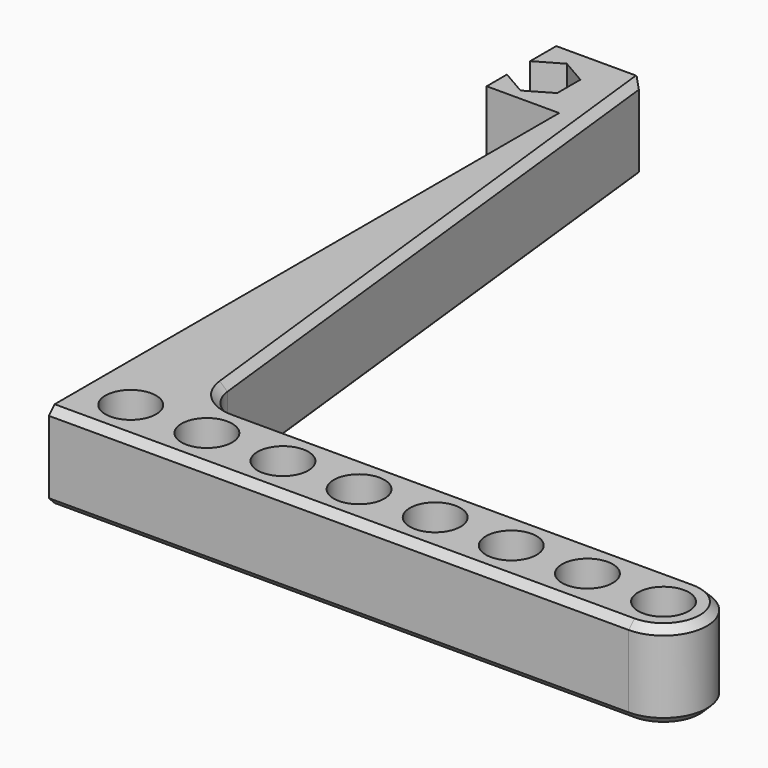
from build123d import *

# Parameters (mm, degrees)
F0_R         = 3.5
F1_DEPTH     = 12
F3_DEPTH     = 25
F4_R         = 5
F5_W         = 12
F5_H         = 12
F6_DEPTH     = 10
F8_T1_DEPTH  = 86.6740446023
F8_T3_DEPTH  = 16.6151120325
F8_T5_DEPTH  = 82.571682988
F8_T7_DEPTH  = 63.5360023124
F8_T10_ANGLE = 180
F8_T12_ANGLE = 83.5169263071
F8_T14_ANGLE = 180
F8_T16_ANGLE = 83.5169263071
F9_DEPTH     = 25


# Not quite as in the source:
# - a fillet or chamfer that OpenCascade refuses, or shapes differently, is made with other operations: its cross-section is extruded or revolved along the edge and cut away or added


with BuildPart() as f1:
    # F0 (on Top) → F1 (new body)
    with BuildSketch(Plane.XY):
        with BuildLine():
            Line((12, 100), (0, 100))
            Line((0, 100), (0, 0))
            Line((0, 0), (80, 0))
            ThreePointArc((80, 0), (86, 6), (80, 12))
            Line((80, 12), (12, 12))
            Line((12, 12), (12, 100))
        make_face()
        with Locations((6.5, 6)):
            Circle(F0_R, mode=Mode.SUBTRACT)
        with Locations((17, 6)):
            Circle(F0_R, mode=Mode.SUBTRACT)
        with Locations((27.5, 6)):
            Circle(F0_R, mode=Mode.SUBTRACT)
        with Locations((38, 6)):
            Circle(F0_R, mode=Mode.SUBTRACT)
        with Locations((48.5, 6)):
            Circle(F0_R, mode=Mode.SUBTRACT)
        with Locations((59, 6)):
            Circle(F0_R, mode=Mode.SUBTRACT)
        with Locations((69.5, 6)):
            Circle(F0_R, mode=Mode.SUBTRACT)
        with Locations((80, 6)):
            Circle(F0_R, mode=Mode.SUBTRACT)
    extrude(amount=F1_DEPTH)

    # F2 (on face) → F3 (cut)
    with BuildSketch(Plane.XY.offset(12)):
        Polygon((2, 100), (12, 12), (12, 100), align=None)
    extrude(amount=-F3_DEPTH, mode=Mode.SUBTRACT)

    # F4
    f4_edges = [f1.edges().sort_by_distance(p)[0] for p in [
        (12, 12, 6),
    ]]
    fillet(f4_edges, radius=F4_R)

    # F5 (on face) → F6 (join)
    with BuildSketch(Plane(origin=(0, 0, 0), x_dir=(0, -1, 0), z_dir=(-1, 0, 0))):
        with Locations((-94, 6)):
            Rectangle(F5_W, F5_H)
    extrude(amount=F6_DEPTH)

    # F8: chamfer of 1 on 11 edges, made by hand

    # F8_s2 → F8_t1 (cut)
    with BuildSketch(Plane(origin=(-11.4836366644, 101.0560026464, 0), x_dir=(0, 0, 1), z_dir=(0.112909688, -0.9936052548, 0))):
        Polygon((12, -12.278179314), (11, -13.278179314), (12, -13.278179314), align=None)
        Polygon((0, -12.278179314), (1, -13.278179314), (0, -13.278179314), align=None)
    extrude(amount=F8_T1_DEPTH, mode=Mode.SUBTRACT)

    # F8_s4 → F8_t3 (cut)
    with BuildSketch(Plane.XY.offset(-2.3075560163)):
        Polygon((1.1072004625, 100), (2.1008057173, 99.112909688), (2, 100), align=None)
    extrude(amount=F8_T3_DEPTH, mode=Mode.SUBTRACT)

    # F8_s6 → F8_t5 (cut)
    with BuildSketch(Plane.YZ.offset(-2.571682988)):
        Polygon((1, 0), (0, 1), (0, 0), align=None)
        Polygon((1, 12), (0, 11), (0, 12), align=None)
    extrude(amount=F8_T5_DEPTH, mode=Mode.SUBTRACT)

    # F8_s8 → F8_t7 (cut)
    with BuildSketch(Plane.YZ.offset(16.4639976876)):
        Polygon((11, 0), (12, 1), (12, 0), align=None)
        Polygon((11, 12), (12, 11), (12, 12), align=None)
    extrude(amount=F8_T7_DEPTH, mode=Mode.SUBTRACT)

    # F8_s9 → F8_t10 (revolve, cut)
    with BuildSketch(Plane.YZ.offset(80)):
        Polygon((1, 0), (0, 1), (0, 0), align=None)
    revolve(axis=Axis((80, 6, 0), (0, 0, 1)), revolution_arc=F8_T10_ANGLE, mode=Mode.SUBTRACT)

    # F8_s11 → F8_t12 (revolve, cut)
    with BuildSketch(Plane(origin=(-1.6972973268, 14.9362164756, 0), x_dir=(0, 0, 1), z_dir=(-0.112909688, 0.9936052548, 0))):
        Polygon((0, 12.278179314), (1, 13.278179314), (0, 13.278179314), align=None)
    revolve(axis=Axis((16.4639976876, 17, 0), (0, 0, 1)), revolution_arc=F8_T12_ANGLE, mode=Mode.SUBTRACT)

    # F8_s13 → F8_t14 (revolve, cut)
    with BuildSketch(Plane.YZ.offset(80)):
        Polygon((1, 12), (0, 11), (0, 12), align=None)
    revolve(axis=Axis((80, 6, 12), (0, 0, 1)), revolution_arc=F8_T14_ANGLE, mode=Mode.SUBTRACT)

    # F8_s15 → F8_t16 (revolve, cut)
    with BuildSketch(Plane(origin=(-1.6972973268, 14.9362164756, 0), x_dir=(0, 0, 1), z_dir=(-0.112909688, 0.9936052548, 0))):
        Polygon((12, 12.278179314), (11, 13.278179314), (12, 13.278179314), align=None)
    revolve(axis=Axis((16.4639976876, 17, 12), (0, 0, 1)), revolution_arc=F8_T16_ANGLE, mode=Mode.SUBTRACT)

    # F7 (on face) → F9 (cut)
    with BuildSketch(Plane.XY.offset(12)):
        Polygon((150.627374606, 89.5), (150.627374606, 97.5), (143.6991713757, 101.5), (136.7709681454, 97.5), (136.7709681454, 89.5), (143.6991713757, 85.5), align=None)
        Polygon((-6.536, 89.5), (-3.0718983849, 91.5), (-3.0718983849, 95.5), (-6.536, 97.5), (-10.0001016151, 95.5), (-10.0001016151, 91.5), align=None)
    extrude(amount=-F9_DEPTH, mode=Mode.SUBTRACT)


solid = f1.part
